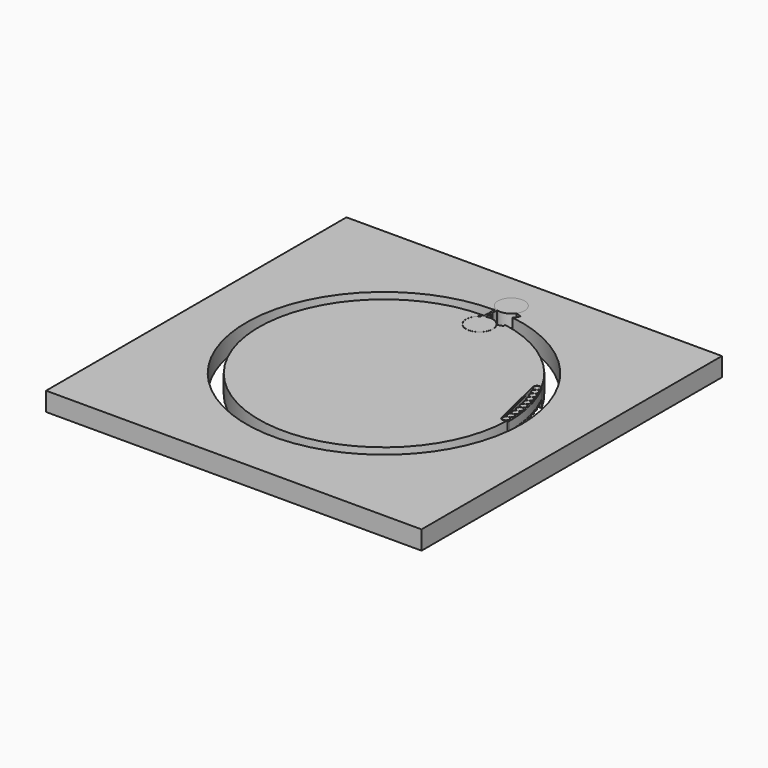
from build123d import *

# Parameters (mm, degrees)
F0_W      = 762
F0_H      = 762
F1_DEPTH  = 38.1
F2_R      = 279.4
F3_DEPTH  = 38.101
F5_DEPTH  = 38.101
F7_START  = -2.54
F7_DEPTH  = 17.78
F8_R      = 6.35
F9_DEPTH  = 25.4
F11_DEPTH = 38.1
F14_DEPTH = 25.4


# Not quite as in the source:
# - a feature of the source that left no trace in its solid (it failed there, or was rolled back) is left out


with BuildPart() as f1:
    # F0 (on Top) → F1 (new body)
    with BuildSketch(Plane.XY):
        Rectangle(F0_W, F0_H)
    extrude(amount=-F1_DEPTH)

    # F2 (on face) → F3 (cut, through all)
    with BuildSketch(Plane.XY):
        Circle(F2_R)
        with BuildLine():
            ThreePointArc((224.3775185155, 119.0408719088), (246.4831532813, 61.3355944662), (254, 0))
            ThreePointArc((254, 0), (253.9910447139, -2.1328865718), (253.9641794872, -4.2656227451))
            ThreePointArc((253.9641794872, -4.2656227451), (-246.9895097327, -59.2636657828), (224.3775185155, 119.0408719088))
        make_face(mode=Mode.SUBTRACT)
    extrude(amount=-F3_DEPTH, mode=Mode.SUBTRACT)

    # F4 (on face) → F5 (cut, through all)
    with BuildSketch(Plane.XY):
        with BuildLine():
            ThreePointArc((224.3775185155, 119.0408719088), (216.0730202223, 118.4392832877), (213.2767121099, 110.5966267409))
            Line((213.2767121099, 110.5966267409), (240.240314708, -1.7779099735))
            ThreePointArc((240.240314708, -1.7779099735), (246.2908782429, -7.4978122175), (253.9641794872, -4.2656227451))
            ThreePointArc((253.9641794872, -4.2656227451), (246.9895097327, 59.2636657828), (224.3775185155, 119.0408719088))
        make_face()
    extrude(amount=-F5_DEPTH, mode=Mode.SUBTRACT)

    # F10 (on face) → F11 (cut, through all)
    with BuildSketch(Plane.XY):
        with BuildLine():
            Line((5.08, 264.5120737159), (0, 264.5120737159))
            Line((0, 264.5120737159), (0, 250.501342462))
            Line((0, 250.501342462), (0, 226.4120737159))
            ThreePointArc((0, 226.4120737159), (2.4632622422, 233.9286686948), (8.8975118233, 238.5294613743))
            Line((8.8975118233, 238.5294613743), (12.615777201, 239.6962689846))
            ThreePointArc((12.615777201, 239.6962689846), (7.1292810208, 244.38136211), (5.08, 251.2988895025))
            Line((5.08, 251.2988895025), (5.08, 264.5120737159))
        make_face()
        with BuildLine():
            ThreePointArc((45.2496747987, 249.9369259045), (25.0130471791, 264.6388819683), (0, 264.5120737159))
            Line((0, 264.5120737159), (5.08, 264.5120737159))
            Line((5.08, 264.5120737159), (5.08, 251.2988895025))
            ThreePointArc((5.08, 251.2988895025), (7.1292810208, 244.38136211), (12.615777201, 239.6962689846))
            Line((12.615777201, 239.6962689846), (45.2496747987, 249.9369259045))
        make_face()
        with BuildLine():
            Line((0, 226.4120737159), (0, 250.501342462))
            ThreePointArc((0, 250.501342462), (5.9898062687, 200.019723142), (35.3633290174, 241.5102983325))
            Line((35.3633290174, 241.5102983325), (34.163640517, 241.1338309397))
            ThreePointArc((34.163640517, 241.1338309397), (27.3570251588, 235.9976267185), (25.3330643469, 227.7142584986))
            ThreePointArc((25.3330643469, 227.7142584986), (25.3832550476, 227.064025706), (25.4, 226.4120737159))
            ThreePointArc((25.4, 226.4120737159), (12.7, 213.7120737159), (0, 226.4120737159))
        make_face()
        with BuildLine():
            Line((46.7706700694, 245.0899708412), (45.2496747987, 249.9369259045))
            Line((45.2496747987, 249.9369259045), (12.615777201, 239.6962689846))
            ThreePointArc((12.615777201, 239.6962689846), (13.9050170211, 239.2044896864), (15.24, 238.8554816092))
            ThreePointArc((15.24, 238.8554816092), (22.1120764722, 234.938668375), (25.3330643469, 227.7142584986))
            ThreePointArc((25.3330643469, 227.7142584986), (27.3570251588, 235.9976267185), (34.163640517, 241.1338309397))
            Line((34.163640517, 241.1338309397), (35.3633290174, 241.5102983325))
            Line((35.3633290174, 241.5102983325), (46.7706700694, 245.0899708412))
        make_face()
        with BuildLine():
            Line((0, 306.9879262841), (0, 268.8879262841))
            ThreePointArc((0, 268.8879262841), (25.0130471791, 268.7611180317), (45.2496747987, 283.4630740955))
            Line((45.2496747987, 283.4630740955), (46.7706700694, 288.3100291588))
            Line((46.7706700694, 288.3100291588), (34.163640517, 292.2661690603))
            ThreePointArc((34.163640517, 292.2661690603), (27.3570251588, 297.4023732815), (25.3330643469, 305.6857415014))
            ThreePointArc((25.3330643469, 305.6857415014), (12.0480480098, 294.3046712365), (0, 306.9879262841))
        make_face()
        with BuildLine():
            ThreePointArc((25.4, 306.9879262841), (12.7, 319.6879262841), (0, 306.9879262841))
            ThreePointArc((0, 306.9879262841), (12.0480480098, 294.3046712365), (25.3330643469, 305.6857415014))
            ThreePointArc((25.3330643469, 305.6857415014), (25.3832550476, 306.335974294), (25.4, 306.9879262841))
        make_face()
        with BuildLine():
            ThreePointArc((15.24, 238.8554816092), (13.9050170211, 239.2044896864), (12.615777201, 239.6962689846))
            Line((12.615777201, 239.6962689846), (8.8975118233, 238.5294613743))
            ThreePointArc((8.8975118233, 238.5294613743), (12.0480480098, 239.0953287635), (15.24, 238.8554816092))
        make_face()
        with BuildLine():
            ThreePointArc((8.8975118233, 238.5294613743), (2.4632622422, 233.9286686948), (0, 226.4120737159))
            ThreePointArc((0, 226.4120737159), (12.7, 213.7120737159), (25.4, 226.4120737159))
            ThreePointArc((25.4, 226.4120737159), (25.3832550476, 227.064025706), (25.3330643469, 227.7142584986))
            ThreePointArc((25.3330643469, 227.7142584986), (22.1120764722, 234.938668375), (15.24, 238.8554816092))
            ThreePointArc((15.24, 238.8554816092), (12.0480480098, 239.0953287635), (8.8975118233, 238.5294613743))
        make_face()
    extrude(amount=-F11_DEPTH, mode=Mode.SUBTRACT)


with BuildPart() as f7:
    # F6 (on face) → F7 (new body)
    with BuildSketch(Plane.XY.offset(F7_START)):
        with BuildLine():
            Line((214.0176806391, 110.7744177383), (240.9812832372, -1.6001189761))
            ThreePointArc((240.9812832372, -1.6001189761), (248.4556377725, -6.8105147955), (254.508, 0))
            ThreePointArc((254.508, 0), (247.4834887521, 59.3821931143), (226.7977130223, 115.4864469619))
            ThreePointArc((226.7977130223, 115.4864469619), (218.3139558622, 118.8091062525), (214.0176806391, 110.7744177383))
        make_face()
        with BuildLine():
            ThreePointArc((254, 0), (248.3959609004, -6.306032218), (241.4752622567, -1.4815916446))
            Line((241.4752622567, -1.4815916446), (214.5116596586, 110.8929450698))
            ThreePointArc((214.5116596586, 110.8929450698), (218.4896922725, 118.3324714719), (226.3450229763, 115.2559350917))
            ThreePointArc((226.3450229763, 115.2559350917), (246.9895097327, 59.2636657828), (254, 0))
        make_face(mode=Mode.SUBTRACT)
    extrude(amount=-F7_DEPTH)


with BuildPart() as f9:
    # F8 (on face) → F9 (new body)
    with BuildSketch(Plane.XY):
        with Locations((247.65, 0)):
            Circle(F8_R)
    extrude(amount=-F9_DEPTH)


with BuildPart() as f9b:
    # F8 (on face) → F9, piece 2 (new body)
    with BuildSketch(Plane.XY):
        with Locations((247.3109710142, 12.954)):
            Circle(F8_R)
    extrude(amount=-F9_DEPTH)


with BuildPart() as f9c:
    # F8 (on face) → F9, piece 3 (new body)
    with BuildSketch(Plane.XY):
        with Locations((246.2948123077, 25.8725323523)):
            Circle(F8_R)
    extrude(amount=-F9_DEPTH)


with BuildPart() as f9d:
    # F8 (on face) → F9, piece 4 (new body)
    with BuildSketch(Plane.XY):
        with Locations((244.6043060912, 38.7202265183)):
            Circle(F8_R)
    extrude(amount=-F9_DEPTH)


with BuildPart() as f9e:
    # F8 (on face) → F9, piece 5 (new body)
    with BuildSketch(Plane.XY):
        with Locations((242.2440809181, 51.4619059126)):
            Circle(F8_R)
    extrude(amount=-F9_DEPTH)


with BuildPart() as f9f:
    # F8 (on face) → F9, piece 6 (new body)
    with BuildSketch(Plane.XY):
        with Locations((239.2205990111, 64.0626842144)):
            Circle(F8_R)
    extrude(amount=-F9_DEPTH)


with BuildPart() as f9g:
    # F8 (on face) → F9, piece 7 (new body)
    with BuildSketch(Plane.XY):
        with Locations((235.5421385695, 76.488060886)):
            Circle(F8_R)
    extrude(amount=-F9_DEPTH)


with BuildPart() as f9h:
    # F8 (on face) → F9, piece 8 (new body)
    with BuildSketch(Plane.XY):
        with Locations((231.2187711031, 88.704015634)):
            Circle(F8_R)
    extrude(amount=-F9_DEPTH)


with BuildPart() as f9i:
    # F8 (on face) → F9, piece 9 (new body)
    with BuildSketch(Plane.XY):
        with Locations((226.262333857, 100.6771015553)):
            Circle(F8_R)
    extrude(amount=-F9_DEPTH)


with BuildPart() as f9j:
    # F8 (on face) → F9, piece 10 (new body)
    with BuildSketch(Plane.XY):
        with Locations((220.6863974019, 112.3745367144)):
            Circle(F8_R)
    extrude(amount=-F9_DEPTH)


with BuildPart() as f14:
    # F13 (on face) → F14 (new body)
    with BuildSketch(Plane.XY):
        with BuildLine():
            Line((4.826, 254), (4.826, 264.2580737159))
            Line((4.826, 264.2580737159), (0.254, 264.2580737159))
            Line((0.254, 264.2580737159), (0.254, 250.3476247431))
            ThreePointArc((0.254, 250.3476247431), (2.4971679316, 251.3863752429), (4.826, 252.2154386704))
            Line((4.826, 252.2154386704), (4.826, 254))
        make_face()
        with BuildLine():
            ThreePointArc((4.826, 252.2154386704), (2.4971679316, 251.3863752429), (0.254, 250.3476247431))
            Line((0.254, 250.3476247431), (0.254, 226.4120737159))
            ThreePointArc((0.254, 226.4120737159), (13.3389129504, 213.9824837692), (25.0804030599, 227.6882148029))
            ThreePointArc((25.0804030599, 227.6882148029), (21.9238349428, 234.7681364818), (15.1892, 238.6066134513))
            ThreePointArc((15.1892, 238.6066134513), (13.8275173615, 238.9626016901), (12.512492745, 239.4642165743))
            ThreePointArc((12.512492745, 239.4642165743), (6.9162666412, 244.2430115622), (4.826, 251.2988895025))
            Line((4.826, 251.2988895025), (4.826, 252.2154386704))
        make_face()
        with BuildLine():
            Line((0, 226.4120737159), (0, 250.2138282516))
            ThreePointArc((0, 250.2138282516), (-1.1779082604, 203.2773123967), (39.6780191819, 226.4120737159))
            ThreePointArc((39.6780191819, 226.4120737159), (38.5109706705, 234.2611062693), (35.1107963914, 241.4310525122))
            Line((35.1107963914, 241.4310525122), (34.163640517, 241.1338309397))
            ThreePointArc((34.163640517, 241.1338309397), (27.3570251588, 235.9976267185), (25.3330643469, 227.7142584986))
            ThreePointArc((25.3330643469, 227.7142584986), (25.3832550476, 227.064025706), (25.4, 226.4120737159))
            ThreePointArc((25.4, 226.4120737159), (12.7, 213.7120737159), (0, 226.4120737159))
        make_face()
        with BuildLine():
            Line((0.254, 226.4120737159), (0.254, 250.3476247431))
            ThreePointArc((0.254, 250.3476247431), (0.1268220256, 250.2810643649), (0, 250.2138282516))
            Line((0, 250.2138282516), (0, 226.4120737159))
            ThreePointArc((0, 226.4120737159), (12.7, 213.7120737159), (25.4, 226.4120737159))
            ThreePointArc((25.4, 226.4120737159), (25.3832550476, 227.064025706), (25.3330643469, 227.7142584986))
            ThreePointArc((25.3330643469, 227.7142584986), (27.3570251588, 235.9976267185), (34.163640517, 241.1338309397))
            Line((34.163640517, 241.1338309397), (35.1107963914, 241.4310525122))
            ThreePointArc((35.1107963914, 241.4310525122), (22.565502396, 251.5215416802), (6.5067237427, 252.6695840354))
            ThreePointArc((6.5067237427, 252.6695840354), (5.6626974395, 252.4560728644), (4.826, 252.2154386704))
            Line((4.826, 252.2154386704), (4.826, 251.2988895025))
            ThreePointArc((4.826, 251.2988895025), (6.9162666412, 244.2430115622), (12.512492745, 239.4642165743))
            ThreePointArc((12.512492745, 239.4642165743), (13.8275173615, 238.9626016901), (15.1892, 238.6066134513))
            ThreePointArc((15.1892, 238.6066134513), (21.9238349428, 234.7681364818), (25.0804030599, 227.6882148029))
            ThreePointArc((25.0804030599, 227.6882148029), (13.3389129504, 213.9824837692), (0.254, 226.4120737159))
        make_face()
    extrude(amount=-F14_DEPTH)


with BuildPart() as f16_1:
    # F16: instance of F14
    add(f14.part.mirror(Plane(origin=(0, 266.7, 0), x_dir=(-1, 0, 0), z_dir=(0, 1, 0))))


solid = Compound([f1.part, f7.part, f9.part, f9b.part, f9c.part, f9d.part, f9e.part, f9f.part, f9g.part, f9h.part, f9i.part, f9j.part, f14.part, f16_1.part])
